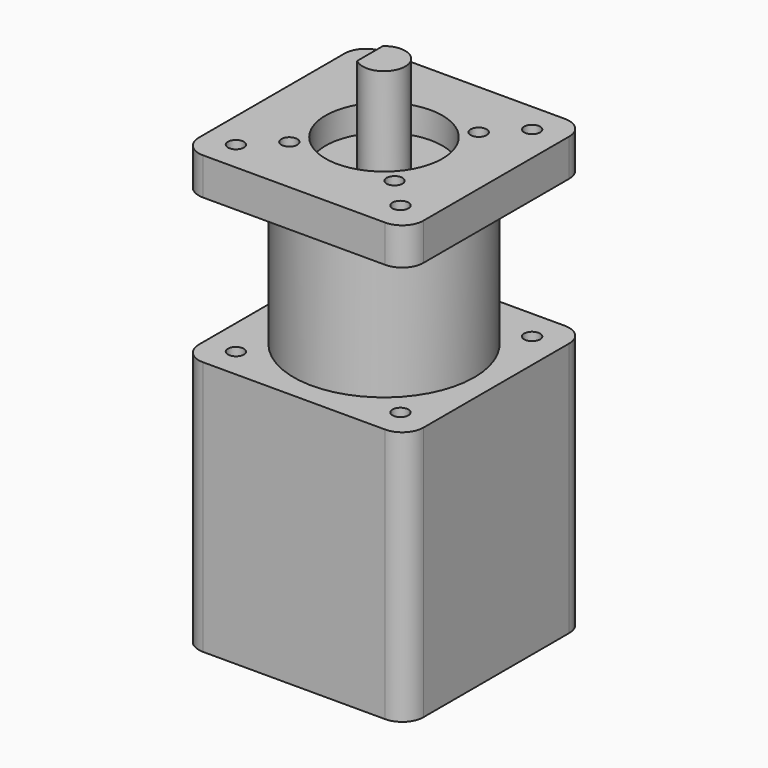
from build123d import *

# Parameters (mm, degrees)
F0_R      = 1.5
F0_R_2    = 17
F0_R_3    = 11
F1_DEPTH  = 7
F2_DEPTH  = 20
F3_DEPTH  = 2
F3_FACE_R = 11
F4_DEPTH  = 75.3
F5_DEPTH  = 27.3
F6_DEPTH  = 35


with BuildPart() as f1:
    # F0 (on Top) → F1 (new body)
    with BuildSketch(Plane.XY):
        with BuildLine():
            ThreePointArc((-21.15, -17.15), (-19.9784271247, -19.9784271247), (-17.15, -21.15))
            Line((-17.15, -21.15), (17.15, -21.15))
            ThreePointArc((17.15, -21.15), (19.9784271247, -19.9784271247), (21.15, -17.15))
            Line((21.15, -17.15), (21.15, 17.15))
            ThreePointArc((21.15, 17.15), (19.9784271247, 19.9784271247), (17.15, 21.15))
            Line((17.15, 21.15), (-17.15, 21.15))
            ThreePointArc((-17.15, 21.15), (-19.9784271247, 19.9784271247), (-21.15, 17.15))
            Line((-21.15, 17.15), (-21.15, -17.15))
        make_face()
        with Locations((-15.4891740419, -15.4891740419)):
            Circle(F0_R, mode=Mode.SUBTRACT)
        with Locations((15.4891740419, -15.4891740419)):
            Circle(F0_R, mode=Mode.SUBTRACT)
        Circle(F0_R_2, mode=Mode.SUBTRACT)
        with Locations((-15.4891740419, 15.4891740419)):
            Circle(F0_R, mode=Mode.SUBTRACT)
        with Locations((15.4891740419, 15.4891740419)):
            Circle(F0_R, mode=Mode.SUBTRACT)
        Circle(F0_R_2)
        with Locations((-9.8994949366, -9.8994949366)):
            Circle(F0_R, mode=Mode.SUBTRACT)
        with Locations((9.8994949366, -9.8994949366)):
            Circle(F0_R, mode=Mode.SUBTRACT)
        Circle(F0_R_3, mode=Mode.SUBTRACT)
        with Locations((-9.8994949366, 9.8994949366)):
            Circle(F0_R, mode=Mode.SUBTRACT)
        with Locations((9.8994949366, 9.8994949366)):
            Circle(F0_R, mode=Mode.SUBTRACT)
    extrude(amount=F1_DEPTH)


with BuildPart() as f2:
    # F0 (on Top) → F2 (new body)
    with BuildSketch(Plane.XY):
        with BuildLine():
            Line((-2.627499033, 3.0159988116), (-2.627499033, -3.0159988116))
            ThreePointArc((-2.627499033, -3.0159988116), (4, 0), (-2.627499033, 3.0159988116))
        make_face()
    extrude(amount=F2_DEPTH)

    # F0 (on Top) → F3 (join)
    with BuildSketch(Plane.XY):
        Circle(F0_R_3)
        with BuildLine():
            ThreePointArc((-2.627499033, 3.0159988116), (4, 0), (-2.627499033, -3.0159988116))
            Line((-2.627499033, -3.0159988116), (-2.627499033, 3.0159988116))
        make_face(mode=Mode.SUBTRACT)
    extrude(amount=F3_DEPTH)

    # F0 (on Top) + F3_face (on face) → F4 (join)
    with BuildSketch(Plane.XY):
        with BuildLine():
            ThreePointArc((-21.15, -17.15), (-19.9784271247, -19.9784271247), (-17.15, -21.15))
            Line((-17.15, -21.15), (17.15, -21.15))
            ThreePointArc((17.15, -21.15), (19.9784271247, -19.9784271247), (21.15, -17.15))
            Line((21.15, -17.15), (21.15, 17.15))
            ThreePointArc((21.15, 17.15), (19.9784271247, 19.9784271247), (17.15, 21.15))
            Line((17.15, 21.15), (-17.15, 21.15))
            ThreePointArc((-17.15, 21.15), (-19.9784271247, 19.9784271247), (-21.15, 17.15))
            Line((-21.15, 17.15), (-21.15, -17.15))
        make_face()
        with Locations((-15.4891740419, -15.4891740419)):
            Circle(F0_R, mode=Mode.SUBTRACT)
        with Locations((15.4891740419, -15.4891740419)):
            Circle(F0_R, mode=Mode.SUBTRACT)
        Circle(F0_R_2, mode=Mode.SUBTRACT)
        with Locations((-15.4891740419, 15.4891740419)):
            Circle(F0_R, mode=Mode.SUBTRACT)
        with Locations((15.4891740419, 15.4891740419)):
            Circle(F0_R, mode=Mode.SUBTRACT)
        Circle(F0_R_2)
        with Locations((-9.8994949366, -9.8994949366)):
            Circle(F0_R, mode=Mode.SUBTRACT)
        with Locations((9.8994949366, -9.8994949366)):
            Circle(F0_R, mode=Mode.SUBTRACT)
        Circle(F0_R_3, mode=Mode.SUBTRACT)
        with Locations((-9.8994949366, 9.8994949366)):
            Circle(F0_R, mode=Mode.SUBTRACT)
        with Locations((9.8994949366, 9.8994949366)):
            Circle(F0_R, mode=Mode.SUBTRACT)
        Circle(F0_R_3)
        with BuildLine():
            ThreePointArc((-2.627499033, 3.0159988116), (4, 0), (-2.627499033, -3.0159988116))
            Line((-2.627499033, -3.0159988116), (-2.627499033, 3.0159988116))
        make_face(mode=Mode.SUBTRACT)
        with BuildLine():
            Line((-2.627499033, 3.0159988116), (-2.627499033, -3.0159988116))
            ThreePointArc((-2.627499033, -3.0159988116), (4, 0), (-2.627499033, 3.0159988116))
        make_face()
        with Locations((15.4891740419, 15.4891740419)):
            Circle(F0_R)
        with Locations((9.8994949366, -9.8994949366)):
            Circle(F0_R)
        with Locations((-15.4891740419, 15.4891740419)):
            Circle(F0_R)
        with Locations((-9.8994949366, 9.8994949366)):
            Circle(F0_R)
        with Locations((15.4891740419, -15.4891740419)):
            Circle(F0_R)
        with Locations((9.8994949366, 9.8994949366)):
            Circle(F0_R)
        with Locations((-9.8994949366, -9.8994949366)):
            Circle(F0_R)
        with Locations((-15.4891740419, -15.4891740419)):
            Circle(F0_R)
    with BuildSketch(Plane(origin=(0, 0, 0), x_dir=(1, 0, 0), z_dir=(0, 0, -1))):
        Circle(F3_FACE_R)
    extrude(amount=-F4_DEPTH, dir=(0, 0, 1))

    # F0 (on Top) → F5 (cut)
    with BuildSketch(Plane.XY):
        with BuildLine():
            ThreePointArc((-21.15, -17.15), (-19.9784271247, -19.9784271247), (-17.15, -21.15))
            Line((-17.15, -21.15), (17.15, -21.15))
            ThreePointArc((17.15, -21.15), (19.9784271247, -19.9784271247), (21.15, -17.15))
            Line((21.15, -17.15), (21.15, 17.15))
            ThreePointArc((21.15, 17.15), (19.9784271247, 19.9784271247), (17.15, 21.15))
            Line((17.15, 21.15), (-17.15, 21.15))
            ThreePointArc((-17.15, 21.15), (-19.9784271247, 19.9784271247), (-21.15, 17.15))
            Line((-21.15, 17.15), (-21.15, -17.15))
        make_face()
        with Locations((-15.4891740419, -15.4891740419)):
            Circle(F0_R, mode=Mode.SUBTRACT)
        with Locations((15.4891740419, -15.4891740419)):
            Circle(F0_R, mode=Mode.SUBTRACT)
        Circle(F0_R_2, mode=Mode.SUBTRACT)
        with Locations((-15.4891740419, 15.4891740419)):
            Circle(F0_R, mode=Mode.SUBTRACT)
        with Locations((15.4891740419, 15.4891740419)):
            Circle(F0_R, mode=Mode.SUBTRACT)
        with Locations((15.4891740419, -15.4891740419)):
            Circle(F0_R)
        with Locations((15.4891740419, 15.4891740419)):
            Circle(F0_R)
        with Locations((9.8994949366, 9.8994949366)):
            Circle(F0_R)
        with Locations((9.8994949366, -9.8994949366)):
            Circle(F0_R)
        with Locations((-9.8994949366, -9.8994949366)):
            Circle(F0_R)
        with Locations((-9.8994949366, 9.8994949366)):
            Circle(F0_R)
        with Locations((-15.4891740419, 15.4891740419)):
            Circle(F0_R)
        with Locations((-15.4891740419, -15.4891740419)):
            Circle(F0_R)
    extrude(amount=-F5_DEPTH, mode=Mode.SUBTRACT)

    # F0 (on Top) → F6 (cut)
    with BuildSketch(Plane.XY):
        with Locations((15.4891740419, -15.4891740419)):
            Circle(F0_R)
        with Locations((-15.4891740419, 15.4891740419)):
            Circle(F0_R)
        with Locations((15.4891740419, 15.4891740419)):
            Circle(F0_R)
        with Locations((-15.4891740419, -15.4891740419)):
            Circle(F0_R)
    extrude(amount=-F6_DEPTH, mode=Mode.SUBTRACT)


solid = Compound([f1.part, f2.part])
